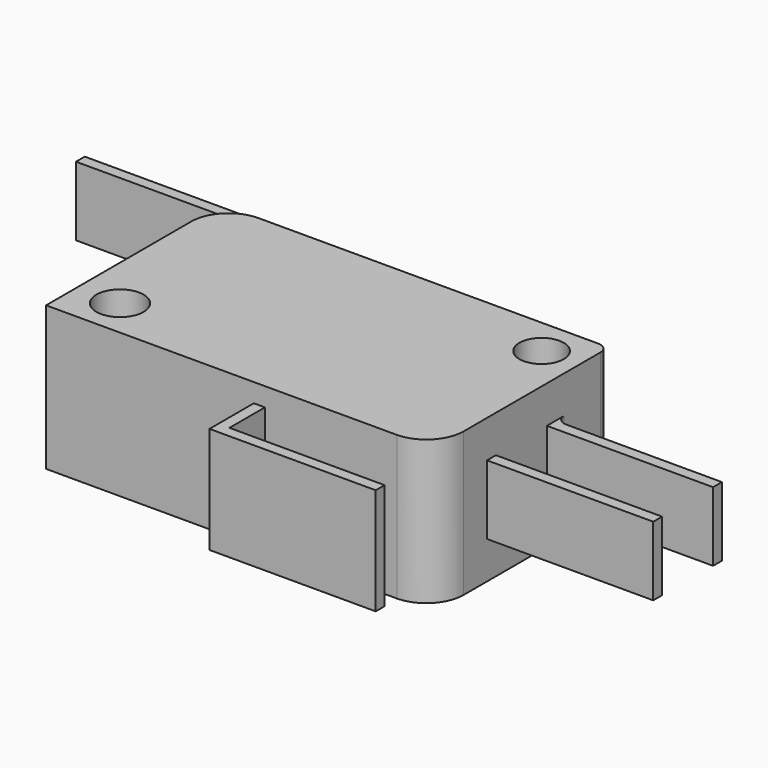
from build123d import *

# Parameters (mm, degrees)
F0_R          = 1.7
F0_R_2        = 1.6
F1_DEPTH      = 10.4
F2_W          = 12.7
F2_H          = 2.7
F2_W_2        = 4
F2_H_2        = 1.35
F3_DEPTH      = 28
F3_DEPTH_BACK = 12.8778
F4_W          = 12
F4_H          = 2.7
F5_DEPTH      = 6.2
F6_T1_DEPTH   = 23.9048285752
F7_R          = 0.762


# Not quite as in the source:
# - a fillet or chamfer that OpenCascade refuses, or shapes differently, is made with other operations: its cross-section is extruded or revolved along the edge and cut away or added
# - a feature names something its author has since deleted; it is built from what else it names


with BuildPart() as f1:
    # F0 (on Top) → F1 (new body)
    with BuildSketch(Plane.XY):
        with BuildLine():
            Line((3.3782, 0), (0, 0))
            Line((0, 0), (0, -15.8))
            Line((0, -15.8), (15, -15.8))
            Line((15, -15.8), (15, -19.8))
            Line((15, -19.8), (27, -19.8))
            Line((27, -19.8), (27, -19))
            Line((27, -19), (15.8, -19))
            Line((15.8, -19), (15.8, -15.8))
            Line((15.8, -15.8), (28, -15.8))
            Line((28, -15.8), (28, -11))
            Line((28, -11), (40, -11))
            Line((40, -11), (40, -10.2))
            Line((40, -10.2), (28, -10.2))
            Line((28, -10.2), (28, -5.6))
            Line((28, -5.6), (40, -5.6))
            Line((40, -5.6), (40, -4.8))
            Line((40, -4.8), (28, -4.8))
            Line((28, -4.8), (28, 0))
            Line((28, 0), (13.31595, 0))
            Line((13.31595, 0), (13.31595, 3.78975))
            Line((13.31595, 3.78975), (-12.8778, 3.78975))
            Line((-12.8778, 3.78975), (-12.8778, 2.996))
            Line((-12.8778, 2.996), (12.5222, 2.996))
            Line((12.5222, 2.996), (12.5222, 0))
            Line((12.5222, 0), (6.1722, 0))
            Line((6.1722, 0), (6.1722, 1.345))
            ThreePointArc((6.1722, 1.345), (4.7752, 2.742), (3.3782, 1.345))
            Line((3.3782, 1.345), (3.3782, 0))
        make_face()
        with Locations((3.1, -13)):
            Circle(F0_R, mode=Mode.SUBTRACT)
        with Locations((25.3, -2.7)):
            Circle(F0_R_2, mode=Mode.SUBTRACT)
    extrude(amount=F1_DEPTH)

    # F2 (on face) → F3 (cut, two sides)
    with BuildSketch(Plane(origin=(0, 0, 0), x_dir=(0, -1, 0), z_dir=(-1, 0, 0))) as f3_sk:
        with Locations((-6.35, 9.05)):
            Rectangle(F2_W, F2_H)
        with Locations((-6.35, 1.35)):
            Rectangle(F2_W, F2_H)
        with Locations((17.8, 9.725)):
            Rectangle(F2_W_2, F2_H_2)
        with Locations((17.8, 0.675)):
            Rectangle(F2_W_2, F2_H_2)
    extrude(amount=-F3_DEPTH, mode=Mode.SUBTRACT)
    extrude(f3_sk.sketch, amount=F3_DEPTH_BACK, mode=Mode.SUBTRACT)

    # F4 (on face) → F5 (cut, through all)
    with BuildSketch(Plane(origin=(0, -4.8, 0), x_dir=(-1, 0, 0), z_dir=(0, 1, 0))):
        with Locations((-34, 9.05)):
            Rectangle(F4_W, F4_H)
        with Locations((-34, 1.35)):
            Rectangle(F4_W, F4_H)
    extrude(amount=-F5_DEPTH, mode=Mode.SUBTRACT)

    # F6: fillet of radius 2.7 on 3 edges, made by hand

    # F6_s2 → F6_t1 (cut)
    with BuildSketch(Plane.XY.offset(-6.7524142876)):
        with BuildLine():
            ThreePointArc((25.2990343146, -15.8004), (27.2091883092, -15.0091883092), (28.0004, -13.0990343146))
            Line((28.0004, -13.0990343146), (28.2705365685, -13.0990343146))
            ThreePointArc((28.2705365685, -13.0990343146), (28.2701365685, -14.4495171573), (28.2701365685, -15.8))
            Line((28.2701365685, -15.8), (28, -16.0701365685))
            ThreePointArc((28, -16.0701365685), (26.6495171573, -16.0701365685), (25.2990343146, -16.0705365685))
            Line((25.2990343146, -16.0705365685), (25.2990343146, -15.8004))
        make_face()
        with BuildLine():
            ThreePointArc((2.7009656854, 0.0004), (0.7908116908, -0.7908116908), (-0.0004, -2.7009656854))
            Line((-0.0004, -2.7009656854), (-0.2705365685, -2.7009656854))
            ThreePointArc((-0.2705365685, -2.7009656854), (-0.2701365685, -1.3504828427), (-0.2701365685, 0))
            Line((-0.2701365685, 0), (0, 0.2701365685))
            ThreePointArc((0, 0.2701365685), (1.3504828427, 0.2701365685), (2.7009656854, 0.2705365685))
            Line((2.7009656854, 0.2705365685), (2.7009656854, 0.0004))
        make_face()
    extrude(amount=F6_T1_DEPTH, mode=Mode.SUBTRACT)

    # F7
    f7_edges = [f1.edges().sort_by_distance(p)[0] for p in [
        (28, 0, 5.2),
        (28, -4.8, 5.2),
    ]]
    fillet(f7_edges, radius=F7_R)


solid = f1.part
